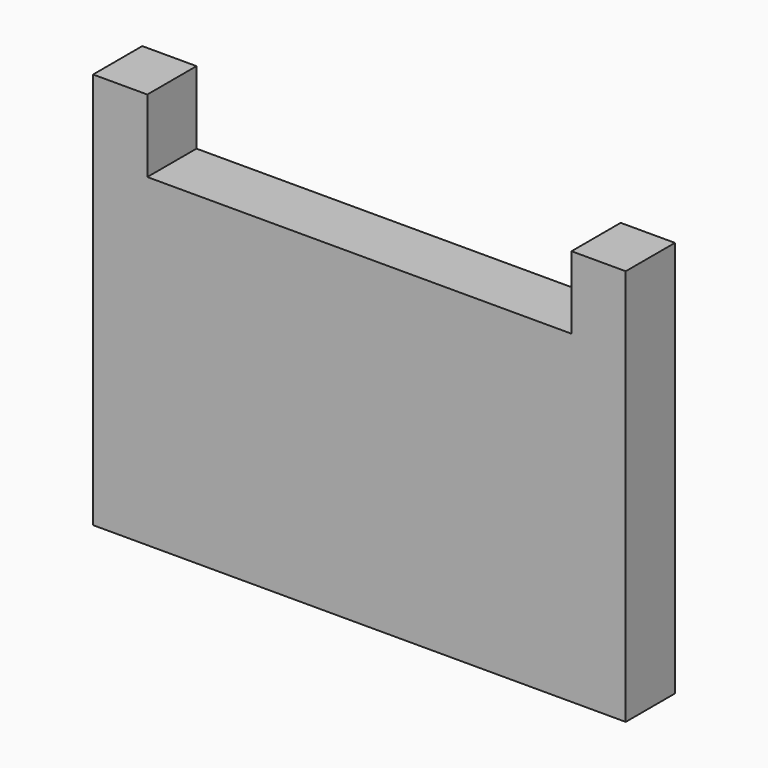
from build123d import *

# Parameters (mm, degrees)
F0_W     = 220
F0_H     = 163.86598641
F1_DEPTH = 25.4
F2_W     = 175.2
F2_H     = 30
F3_DEPTH = 57.15


# Not quite as in the source:
# - a feature names something its author has since deleted; it is built from what else it names


with BuildPart() as f1:
    # F0 (on Front) → F1 (new body)
    with BuildSketch(Plane.XZ):
        with Locations((1.3140309602, -1.7520450056)):
            Rectangle(F0_W, F0_H)
    extrude(amount=F1_DEPTH)

    # F2 (on face) → F3 (cut)
    with BuildSketch(Plane.XZ.offset(25.4)):
        with Locations((1.3140309602, 65.1809481994)):
            Rectangle(F2_W, F2_H)
    extrude(amount=-F3_DEPTH, mode=Mode.SUBTRACT)


solid = f1.part
